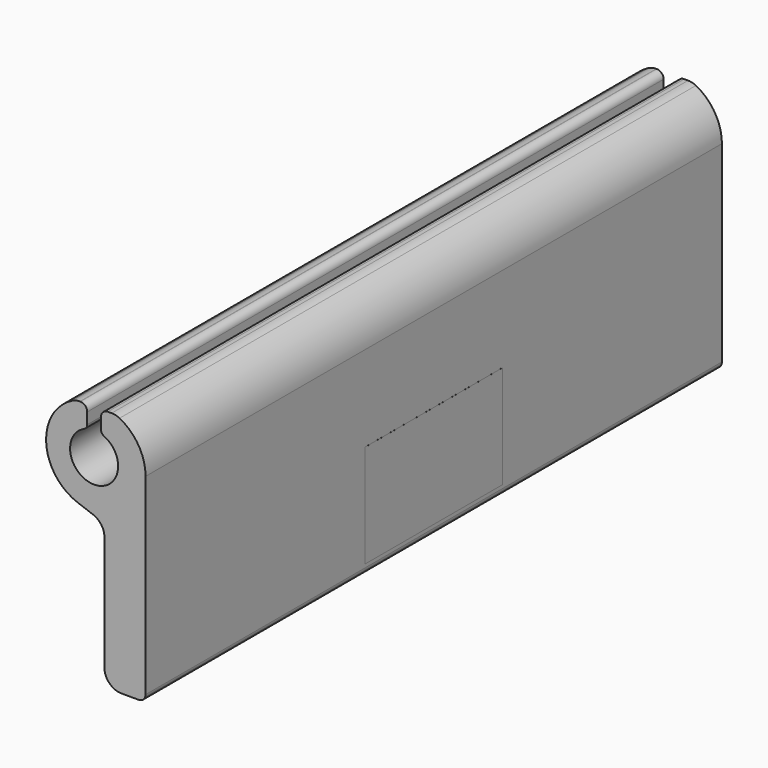
from build123d import *

# Parameters (mm, degrees)
F1_DEPTH = 105
F2_R     = 12
F3_DEPTH = 0.05
F4_W     = 50
F4_H     = 30
F5_DEPTH = 0.01


# Not quite as in the source:
# - ends of sketch curves that miss each other by under 0.0002 mm in the source are joined


with BuildPart() as f1:
    # F0 (on Front) → F1 (new body, symmetric)
    with BuildSketch(Plane.XZ):
        with BuildLine():
            Line((2.4999997663, 3.0085625581), (2.4999997663, -30.5))
            ThreePointArc((2.4999997663, -30.5), (3.9644658603, -34.0355339059), (7.4999997663, -35.5))
            Line((7.4999997663, -35.5), (12.4999997663, -35.5))
            ThreePointArc((12.4999997663, -35.5), (13.9142133287, -34.9142135624), (14.4999997663, -33.5))
            Line((14.4999997663, -33.5), (14.4999997663, 22.4999994828))
            ThreePointArc((14.4999997663, 22.4999994828), (12.4539129776, 29.7872458033), (6.9137199183, 34.9444437777))
            ThreePointArc((6.9137199183, 34.9444437777), (5.8016169865, 35.3591259101), (4.6231056877, 35.4999993303))
            Line((4.6231056877, 35.4999993303), (3.4999997663, 35.4999993303))
            ThreePointArc((3.4999997663, 35.4999993303), (2.0857862039, 34.9142128927), (1.4999997663, 33.4999993303))
            Line((1.4999997663, 33.4999993303), (1.4999997663, 30.2459664828))
            ThreePointArc((1.4999997663, 30.2459664828), (1.7397477835, 29.4324771221), (2.3823530195, 28.8790310431))
            ThreePointArc((2.3823530195, 28.8790310431), (-0.5000000985, 15.4999997293), (-3.3823532363, 28.8790310342))
            ThreePointArc((-3.3823532363, 28.8790310342), (-2.7397478169, 29.4324771961), (-2.4999997997, 30.2459665567))
            Line((-2.4999997997, 30.2459665567), (-2.4999997997, 33.5))
            ThreePointArc((-2.4999997997, 33.5), (-3.0857862373, 34.9142132361), (-4.4999997997, 35.4999996738))
            Line((-4.4999997997, 35.4999996738), (-4.6231058319, 35.4999996738))
            ThreePointArc((-4.6231058319, 35.4999996738), (-5.8016171306, 35.3591262536), (-6.9137200625, 34.9444441212))
            ThreePointArc((-6.9137200625, 34.9444441212), (-14.4718653147, 21.6128794539), (-5.288282, 9.344303))
            Line((-5.288282, 9.344303), (-0.7898995061, 7.707025658))
            ThreePointArc((-0.7898995061, 7.707025658), (1.5957599911, 5.8764447351), (2.4999997663, 3.0085625581))
        make_face()
    extrude(amount=F1_DEPTH, both=True)

    # F2 (on face) → F3 (join)
    with BuildSketch(Plane(origin=(2.4999997663, 0, 0), x_dir=(0, -1, 0), z_dir=(-1, 0, 0))):
        with Locations((0, -11.5)):
            Circle(F2_R)
    extrude(amount=F3_DEPTH)

    # F4 (on face) → F5 (join)
    with BuildSketch(Plane.YZ.offset(14.4999997663)):
        with Locations((0, -17.5000005172)):
            Rectangle(F4_W, F4_H)
    extrude(amount=F5_DEPTH)


solid = f1.part
